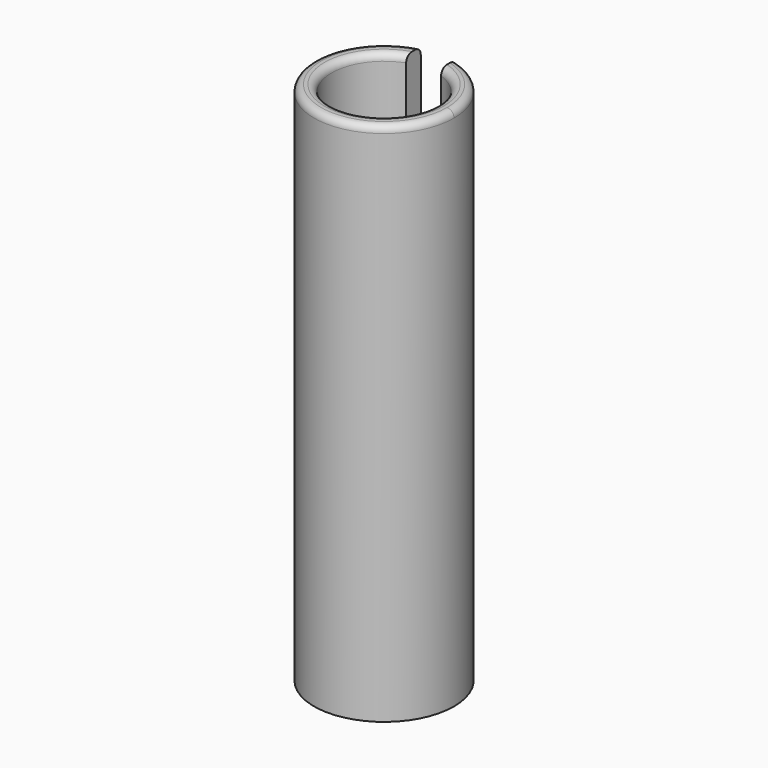
from build123d import *

# Parameters (mm, degrees)
F0_R     = 10
F0_R_2   = 7.5
F1_DEPTH = 45
F2_DEPTH = 5
F3_R     = 10
F3_R_2   = 8.4
F4_DEPTH = 30
F5_SIZE  = 2
F6_W     = 5
F6_H     = 16.3043601838
F7_DEPTH = 35
F8_R     = 2
F9_R     = 1


with BuildPart() as f1:
    # F0 (on Top) → F1 (new body)
    with BuildSketch(Plane.XY):
        Circle(F0_R)
        Circle(F0_R_2, mode=Mode.SUBTRACT)
    extrude(amount=F1_DEPTH)

    # F0 (on Top) → F2 (join)
    with BuildSketch(Plane.XY):
        Circle(F0_R)
        Circle(F0_R_2, mode=Mode.SUBTRACT)
        Circle(F0_R_2)
    extrude(amount=F2_DEPTH)

    # F3 (on Top) + F0 (on Top) → F4 (join)
    with BuildSketch(Plane.XY):
        Circle(F3_R)
        Circle(F3_R_2, mode=Mode.SUBTRACT)
    with BuildSketch(Plane.XY):
        Circle(F0_R_2)
    extrude(amount=-F4_DEPTH)

    # F5
    f5_edges = [f1.edges().sort_by_distance(p)[0] for p in [
        (-7.5, 0, -30),
    ]]
    chamfer(f5_edges, length=F5_SIZE)

    # F6 (on face) → F7 (cut)
    with BuildSketch(Plane.XY.offset(45)):
        with Locations((0, 8.1521800919)):
            Rectangle(F6_W, F6_H)
    extrude(amount=-F7_DEPTH, mode=Mode.SUBTRACT)

    # F8
    f8_edges = [f1.edges().sort_by_distance(p)[0] for p in [
        (2.5, 8.376763, 10),
        (-2.5, 8.376763, 10),
    ]]
    fillet(f8_edges, radius=F8_R)

    # F9
    f9_edges = [f1.edges().sort_by_distance(p)[0] for p in [
        (-6.123724, -7.905694, 45),
        (7.905694, 6.123724, 45),
        (-4.330127, -6.123724, 45),
        (6.123724, 4.330127, 45),
    ]]
    fillet(f9_edges, radius=F9_R)


solid = f1.part
